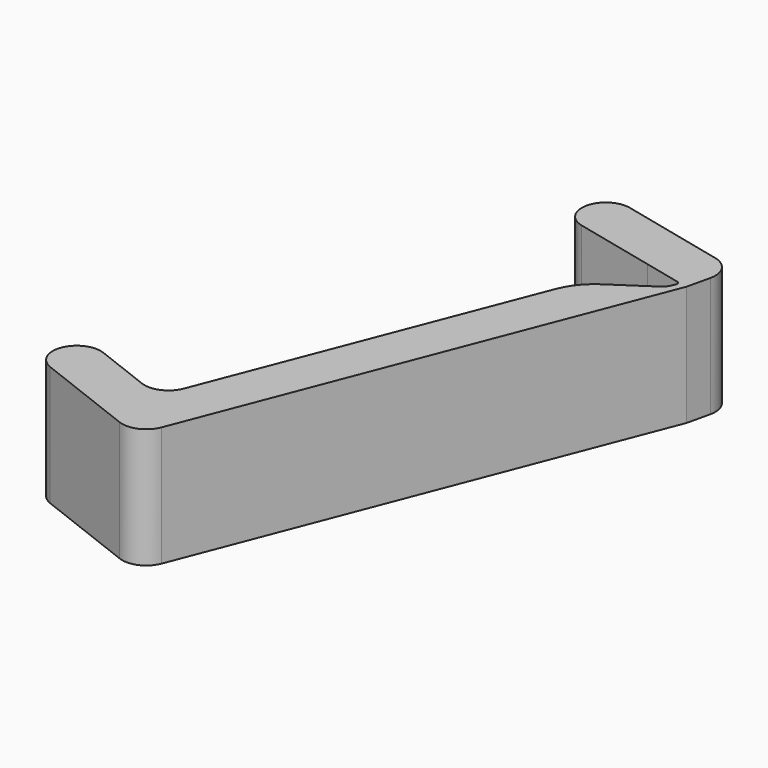
from build123d import *

# Parameters (mm, degrees)
F1_DEPTH     = 20
F2_TEXT_SIZE = 5.5555555556
F3_DEPTH     = 1
F4_R         = 3.99999
F5_R         = 10
F6_R         = 0.5
F7_R         = 3
F8_T1_DEPTH  = 40
F8_T3_DEPTH  = 39.9414494705


# Not quite as in the source:
# - a fillet or chamfer that OpenCascade refuses, or shapes differently, is made with other operations: its cross-section is extruded or revolved along the edge and cut away or added
# - a fillet or chamfer is up to 0.001 mm smaller than in the source, because OpenCascade refuses the exact size
# - Text() gives the source's letters only with a copy of the font that has no kerning and outlines rounded to 1/6400 em; it was checked with that copy


with BuildPart() as f1:
    # F0 (on Top) → F1 (new body)
    with BuildSketch(Plane.XY):
        Polygon((4.3357486672, 52.4938509933), (-18.4977839839, -6.3360708644), (-35.2781781601, 0.1768678957), (-38.172817609, -7.2810850714), (-13.9344704657, -16.6886632805), (16.097413817, 60.687598754), (17.8855298351, 68.4053416131), (-7.4262132119, 74.3480399836), (-9.2547357874, 66.5598113537), (8.2041985264, 62.4607976941), (14.8400965361, 60.9028196357), (14.1164366739, 59.0383313939), align=None)
    extrude(amount=F1_DEPTH)

    # F2 (on face) → F3 (cut)
    with BuildSketch(Plane(origin=(16.1555836554, 68.8114988787, 0), x_dir=(-0.9735285787, 0.2285653219, 0), z_dir=(0.2285653219, 0.9735285787, 0))):
        with Locations(Location((23.0249170735, 7.3618779402), (0, 0, 180))):
            Text('10 deg.', F2_TEXT_SIZE, font='Open Sans', font_style=FontStyle.BOLD, text_align=(TextAlign.LEFT, TextAlign.BOTTOM))
        with Locations(Location((23.0249170735, 14.9174334958), (0, 0, 180))):
            Text('1.25 mm', F2_TEXT_SIZE, font='Open Sans', font_style=FontStyle.BOLD, text_align=(TextAlign.LEFT, TextAlign.BOTTOM))
    extrude(amount=-F3_DEPTH, mode=Mode.SUBTRACT)

    # F4 (radius 4 in the source; OpenCascade refuses exactly that, so slightly less here)
    f4_edges = [f1.edges().sort_by_distance(p)[0] for p in [
        (-35.278178, 0.176868, 10),
        (-38.172818, -7.281085, 10),
        (-18.497784, -6.336071, 10),
        (-13.93447, -16.688663, 10),
    ]]
    fillet(f4_edges, radius=F4_R)

    # F5
    f5_edges = [f1.edges().sort_by_distance(p)[0] for p in [
        (4.335749, 52.493851, 10),
    ]]
    fillet(f5_edges, radius=F5_R)

    # F6
    f6_edges = [f1.edges().sort_by_distance(p)[0] for p in [
        (14.840097, 60.90282, 10),
    ]]
    fillet(f6_edges, radius=F6_R)

    # F7
    f7_edges = [f1.edges().sort_by_distance(p)[0] for p in [
        (14.116437, 59.038331, 10),
    ]]
    fillet(f7_edges, radius=F7_R)

    # F8: fillet of radius 4 on 3 edges, made by hand

    # F8_s2 → F8_t1 (cut)
    with BuildSketch(Plane.XY.offset(-10)):
        with BuildLine():
            ThreePointArc((-5.3606214725, 65.645550066), (-7.8463951799, 67.4325900985), (-8.3404744997, 70.4539256687))
            Line((-8.3404744997, 70.4539256687), (-9.2547357874, 66.5598113537))
            Line((-9.2547357874, 66.5598113537), (-5.3606214725, 65.645550066))
        make_face()
        with BuildLine():
            ThreePointArc((-8.3404744997, 70.4539256687), (-6.5534344672, 72.9396993761), (-3.532098897, 73.4337786958))
            Line((-3.532098897, 73.4337786958), (-7.4262132119, 74.3480399836))
            Line((-7.4262132119, 74.3480399836), (-8.3404744997, 70.4539256687))
        make_face()
    extrude(amount=F8_T1_DEPTH, mode=Mode.SUBTRACT)

    # F8_s4 → F8_t3 (cut)
    with BuildSketch(Plane.XY.offset(-9.9707247353)):
        with BuildLine():
            ThreePointArc((14.0028156429, 69.3169263767), (16.4854969214, 67.5348682168), (16.985332376, 64.5199715131))
            Line((16.985332376, 64.5199715131), (17.8855298351, 68.4053416131))
            Line((17.8855298351, 68.4053416131), (14.0028156429, 69.3169263767))
        make_face()
    extrude(amount=F8_T3_DEPTH, mode=Mode.SUBTRACT)


solid = f1.part
